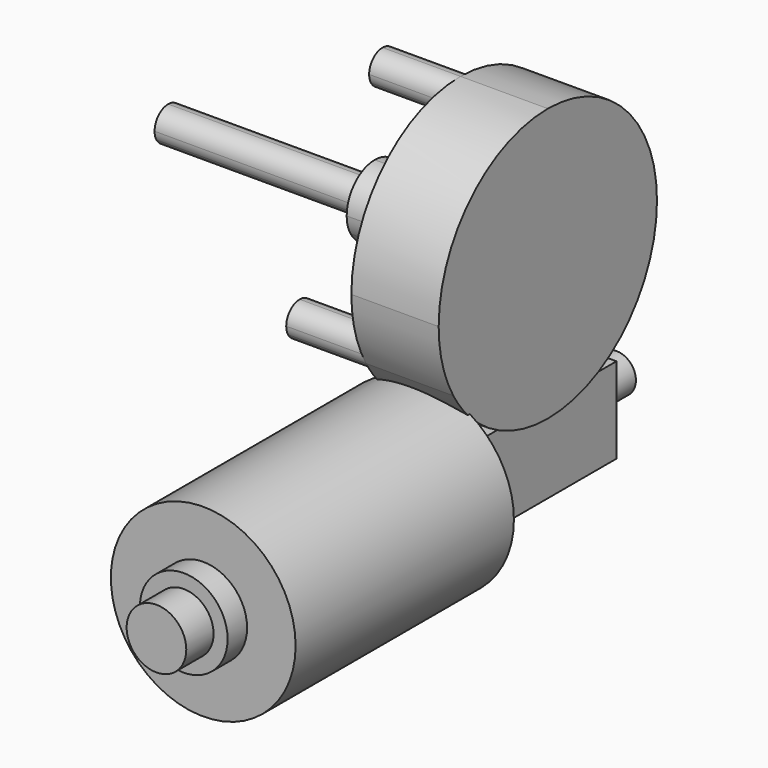
from build123d import *

# Parameters (mm, degrees)
F0_R      = 30.099
F0_R_2    = 14.2875
F0_R_3    = 9.7155
F1_DEPTH  = 88.9
F2_DEPTH  = 7.9375
F3_DEPTH  = 19.05
F4_W      = 25.4
F4_H      = 27.94
F4_R      = 6.35
F5_DEPTH  = 63.5
F6_DEPTH  = 79.375
F8_DEPTH  = 28.448
F9_DEPTH  = 27.94
F10_DEPTH = 95.25
F11_DEPTH = 25.4


# Not quite as in the source:
# - a length typed as a fraction of an inch, garbled in the dataset ("3 / 203.2 mm" for 3/8 in), is restored


with BuildPart() as f1:
    # F0 (on Front) → F1 (new body)
    with BuildSketch(Plane.XZ):
        Circle(F0_R)
        Circle(F0_R_2, mode=Mode.SUBTRACT)
        Circle(F0_R_2)
        Circle(F0_R_3, mode=Mode.SUBTRACT)
        Circle(F0_R_3)
    extrude(amount=-F1_DEPTH)

    # F0 (on Front) → F2 (join)
    with BuildSketch(Plane.XZ):
        Circle(F0_R_2)
        Circle(F0_R_3, mode=Mode.SUBTRACT)
    extrude(amount=F2_DEPTH)

    # F0 (on Front) → F3 (join)
    with BuildSketch(Plane.XZ):
        Circle(F0_R_3)
    extrude(amount=F3_DEPTH)

    # F4 (on face) → F5 (join)
    with BuildSketch(Plane(origin=(0, 88.9, 0), x_dir=(-1, 0, 0), z_dir=(0, 1, 0))):
        Rectangle(F4_W, F4_H)
        Circle(F4_R, mode=Mode.SUBTRACT)
    extrude(amount=F5_DEPTH)

    # F4 (on face) → F6 (join)
    with BuildSketch(Plane(origin=(0, 88.9, 0), x_dir=(-1, 0, 0), z_dir=(0, 1, 0))):
        Circle(F4_R)
    extrude(amount=F6_DEPTH)

    # F7 (on face) → F8 (join)
    with BuildSketch(Plane(origin=(-12.7, 0, 0), x_dir=(0, -1, 0), z_dir=(-1, 0, 0))):
        with BuildLine():
            Line((-120.65, 33.655), (-120.65, 13.97))
            Line((-120.65, 13.97), (-120.65, 11.43))
            ThreePointArc((-120.65, 11.43), (-98.425, 17.3851708018), (-82.1551708018, 33.655))
            ThreePointArc((-82.1551708018, 33.655), (-86.8845355318, 30.9245), (-91.6139002619, 33.655))
            Line((-91.6139002619, 33.655), (-120.65, 33.655))
        make_face()
        with BuildLine():
            Line((-120.65, 11.43), (-120.65, 13.97))
            Line((-120.65, 13.97), (-120.65, 33.655))
            Line((-120.65, 33.655), (-149.6860997381, 33.655))
            ThreePointArc((-149.6860997381, 33.655), (-154.4154644682, 30.9245), (-159.1448291982, 33.655))
            ThreePointArc((-159.1448291982, 33.655), (-142.875, 17.3851708018), (-120.65, 11.43))
        make_face()
        with BuildLine():
            Line((-156.5051837675, 35.179), (-159.1448291982, 33.655))
            Line((-159.1448291982, 33.655), (-149.6860997381, 33.655))
            ThreePointArc((-149.6860997381, 33.655), (-149.1405435308, 34.9720891947), (-148.9544644682, 36.3855))
            ThreePointArc((-148.9544644682, 36.3855), (-149.1405435308, 37.7989108053), (-149.6860997381, 39.116))
            Line((-149.6860997381, 39.116), (-152.3257451688, 37.592))
            ThreePointArc((-152.3257451688, 37.592), (-152.0846854493, 37.0100303558), (-152.0024644682, 36.3855))
            ThreePointArc((-152.0024644682, 36.3855), (-153.7909341123, 34.0547209812), (-156.5051837675, 35.179))
        make_face()
        with BuildLine():
            ThreePointArc((-154.4154644682, 41.8465), (-159.1448291982, 39.116), (-159.1448291982, 33.655))
            Line((-159.1448291982, 33.655), (-154.4154644682, 41.8465))
        make_face()
        with BuildLine():
            Line((-154.4154644682, 41.8465), (-159.1448291982, 33.655))
            Line((-159.1448291982, 33.655), (-156.5051837675, 35.179))
            ThreePointArc((-156.5051837675, 35.179), (-155.6219644682, 38.4752192993), (-152.3257451688, 37.592))
            Line((-152.3257451688, 37.592), (-149.6860997381, 39.116))
            ThreePointArc((-149.6860997381, 39.116), (-151.6849644682, 41.1148647301), (-154.4154644682, 41.8465))
        make_face()
        with BuildLine():
            ThreePointArc((-120.65, 100.33), (-159.1448291982, 78.105), (-159.1448291982, 33.655))
            ThreePointArc((-159.1448291982, 33.655), (-159.1448291982, 39.116), (-154.4154644682, 41.8465))
            Line((-154.4154644682, 41.8465), (-125.3793647301, 92.1385))
            ThreePointArc((-125.3793647301, 92.1385), (-125.3793647301, 97.5995), (-120.65, 100.33))
        make_face()
        with BuildLine():
            Line((-149.6860997381, 33.655), (-159.1448291982, 33.655))
            ThreePointArc((-159.1448291982, 33.655), (-154.4154644682, 30.9245), (-149.6860997381, 33.655))
        make_face()
        with BuildLine():
            ThreePointArc((-81.4235355318, 36.3855), (-81.6096145945, 34.9720891947), (-82.1551708018, 33.655))
            ThreePointArc((-82.1551708018, 33.655), (-77.7145970215, 44.3754934452), (-76.2, 55.88))
            ThreePointArc((-76.2, 55.88), (-89.2191035763, 87.3108964237), (-120.65, 100.33))
            ThreePointArc((-120.65, 100.33), (-116.7884898679, 98.7305101321), (-115.189, 94.869))
            ThreePointArc((-115.189, 94.869), (-115.3750790626, 93.4555891947), (-115.9206352699, 92.1385))
            Line((-115.9206352699, 92.1385), (-86.8845355318, 41.8465))
            ThreePointArc((-86.8845355318, 41.8465), (-83.0230253998, 40.2470101321), (-81.4235355318, 36.3855))
        make_face()
        with BuildLine():
            Line((-84.7948162325, 35.179), (-82.1551708018, 33.655))
            Line((-82.1551708018, 33.655), (-86.8845355318, 41.8465))
            ThreePointArc((-86.8845355318, 41.8465), (-89.6150355318, 41.1148647301), (-91.6139002619, 39.116))
            Line((-91.6139002619, 39.116), (-88.9742548312, 37.592))
            ThreePointArc((-88.9742548312, 37.592), (-86.260005176, 38.7162790188), (-84.4715355318, 36.3855))
            ThreePointArc((-84.4715355318, 36.3855), (-84.553756513, 35.7609696442), (-84.7948162325, 35.179))
        make_face()
        with BuildLine():
            ThreePointArc((-91.6139002619, 33.655), (-86.8845355318, 30.9245), (-82.1551708018, 33.655))
            Line((-82.1551708018, 33.655), (-91.6139002619, 33.655))
        make_face()
        with BuildLine():
            Line((-91.6139002619, 33.655), (-82.1551708018, 33.655))
            Line((-82.1551708018, 33.655), (-84.7948162325, 35.179))
            ThreePointArc((-84.7948162325, 35.179), (-88.0910355318, 34.2957807007), (-88.9742548312, 37.592))
            Line((-88.9742548312, 37.592), (-91.6139002619, 39.116))
            ThreePointArc((-91.6139002619, 39.116), (-92.3455355318, 36.3855), (-91.6139002619, 33.655))
        make_face()
        with BuildLine():
            Line((-86.8845355318, 41.8465), (-82.1551708018, 33.655))
            ThreePointArc((-82.1551708018, 33.655), (-81.6096145945, 34.9720891947), (-81.4235355318, 36.3855))
            ThreePointArc((-81.4235355318, 36.3855), (-83.0230253998, 40.2470101321), (-86.8845355318, 41.8465))
        make_face()
        with BuildLine():
            ThreePointArc((-115.189, 94.869), (-116.7884898679, 98.7305101321), (-120.65, 100.33))
            Line((-120.65, 100.33), (-115.9206352699, 92.1385))
            ThreePointArc((-115.9206352699, 92.1385), (-115.3750790626, 93.4555891947), (-115.189, 94.869))
        make_face()
        with BuildLine():
            Line((-120.65, 97.282), (-120.65, 100.33))
            Line((-120.65, 100.33), (-125.3793647301, 92.1385))
            ThreePointArc((-125.3793647301, 92.1385), (-123.3805, 90.1396352699), (-120.65, 89.408))
            Line((-120.65, 89.408), (-120.65, 92.456))
            ThreePointArc((-120.65, 92.456), (-123.063, 94.869), (-120.65, 97.282))
        make_face()
        with BuildLine():
            Line((-115.9206352699, 92.1385), (-120.65, 100.33))
            Line((-120.65, 100.33), (-120.65, 97.282))
            ThreePointArc((-120.65, 97.282), (-118.943751337, 96.575248663), (-118.237, 94.869))
            ThreePointArc((-118.237, 94.869), (-118.943751337, 93.162751337), (-120.65, 92.456))
            Line((-120.65, 92.456), (-120.65, 89.408))
            ThreePointArc((-120.65, 89.408), (-117.9195, 90.1396352699), (-115.9206352699, 92.1385))
        make_face()
        with BuildLine():
            Line((-125.3793647301, 92.1385), (-120.65, 100.33))
            ThreePointArc((-120.65, 100.33), (-125.3793647301, 97.5995), (-125.3793647301, 92.1385))
        make_face()
        with BuildLine():
            ThreePointArc((-120.65, 67.31), (-130.5486703653, 61.595), (-130.5486703653, 50.165))
            Line((-130.5486703653, 50.165), (-125.4343573432, 53.11775))
            ThreePointArc((-125.4343573432, 53.11775), (-125.4343573432, 58.64225), (-120.65, 61.4045))
            Line((-120.65, 61.4045), (-120.65, 67.31))
        make_face()
        with BuildLine():
            ThreePointArc((-130.5486703653, 50.165), (-126.365, 45.9813296347), (-120.65, 44.45))
            Line((-120.65, 44.45), (-120.65, 50.3555))
            ThreePointArc((-120.65, 50.3555), (-123.41225, 51.0956426568), (-125.4343573432, 53.11775))
            Line((-125.4343573432, 53.11775), (-130.5486703653, 50.165))
        make_face()
        with BuildLine():
            Line((-120.65, 50.3555), (-120.65, 44.45))
            ThreePointArc((-120.65, 44.45), (-114.935, 45.9813296347), (-110.7513296347, 50.165))
            Line((-110.7513296347, 50.165), (-115.8656426568, 53.11775))
            ThreePointArc((-115.8656426568, 53.11775), (-117.88775, 51.0956426568), (-120.65, 50.3555))
        make_face()
        with BuildLine():
            Line((-115.8656426568, 53.11775), (-110.7513296347, 50.165))
            ThreePointArc((-110.7513296347, 50.165), (-109.6094678055, 52.9216983145), (-109.22, 55.88))
            ThreePointArc((-109.22, 55.88), (-112.567769491, 63.962230509), (-120.65, 67.31))
            Line((-120.65, 67.31), (-120.65, 61.4045))
            ThreePointArc((-120.65, 61.4045), (-116.7435885873, 59.7864114127), (-115.1255, 55.88))
            ThreePointArc((-115.1255, 55.88), (-115.3137427727, 54.4501541853), (-115.8656426568, 53.11775))
        make_face()
        with BuildLine():
            Line((-125.4343573432, 53.11775), (-120.65, 55.88))
            Line((-120.65, 55.88), (-120.65, 61.4045))
            ThreePointArc((-120.65, 61.4045), (-125.4343573432, 58.64225), (-125.4343573432, 53.11775))
        make_face()
        with BuildLine():
            ThreePointArc((-125.4343573432, 53.11775), (-123.41225, 51.0956426568), (-120.65, 50.3555))
            Line((-120.65, 50.3555), (-120.65, 55.88))
            Line((-120.65, 55.88), (-125.4343573432, 53.11775))
        make_face()
        with BuildLine():
            Line((-120.65, 55.88), (-120.65, 50.3555))
            ThreePointArc((-120.65, 50.3555), (-117.88775, 51.0956426568), (-115.8656426568, 53.11775))
            Line((-115.8656426568, 53.11775), (-120.65, 55.88))
        make_face()
        with BuildLine():
            Line((-120.65, 61.4045), (-120.65, 55.88))
            Line((-120.65, 55.88), (-115.8656426568, 53.11775))
            ThreePointArc((-115.8656426568, 53.11775), (-115.3137427727, 54.4501541853), (-115.1255, 55.88))
            ThreePointArc((-115.1255, 55.88), (-116.7435885873, 59.7864114127), (-120.65, 61.4045))
        make_face()
        with BuildLine():
            ThreePointArc((-109.22, 55.88), (-109.6094678055, 52.9216983145), (-110.7513296347, 50.165))
            Line((-110.7513296347, 50.165), (-91.6139002619, 39.116))
            ThreePointArc((-91.6139002619, 39.116), (-89.6150355318, 41.1148647301), (-86.8845355318, 41.8465))
            Line((-86.8845355318, 41.8465), (-115.9206352699, 92.1385))
            ThreePointArc((-115.9206352699, 92.1385), (-117.9195, 90.1396352699), (-120.65, 89.408))
            Line((-120.65, 89.408), (-120.65, 67.31))
            ThreePointArc((-120.65, 67.31), (-112.567769491, 63.962230509), (-109.22, 55.88))
        make_face()
        with BuildLine():
            Line((-149.6860997381, 39.116), (-130.5486703653, 50.165))
            ThreePointArc((-130.5486703653, 50.165), (-130.5486703653, 61.595), (-120.65, 67.31))
            Line((-120.65, 67.31), (-120.65, 89.408))
            ThreePointArc((-120.65, 89.408), (-123.3805, 90.1396352699), (-125.3793647301, 92.1385))
            Line((-125.3793647301, 92.1385), (-154.4154644682, 41.8465))
            ThreePointArc((-154.4154644682, 41.8465), (-151.6849644682, 41.1148647301), (-149.6860997381, 39.116))
        make_face()
        with BuildLine():
            Line((-149.6860997381, 33.655), (-120.65, 33.655))
            Line((-120.65, 33.655), (-120.65, 44.45))
            ThreePointArc((-120.65, 44.45), (-126.365, 45.9813296347), (-130.5486703653, 50.165))
            Line((-130.5486703653, 50.165), (-149.6860997381, 39.116))
            ThreePointArc((-149.6860997381, 39.116), (-149.1405435308, 37.7989108053), (-148.9544644682, 36.3855))
            ThreePointArc((-148.9544644682, 36.3855), (-149.1405435308, 34.9720891947), (-149.6860997381, 33.655))
        make_face()
        with BuildLine():
            Line((-120.65, 44.45), (-120.65, 33.655))
            Line((-120.65, 33.655), (-91.6139002619, 33.655))
            ThreePointArc((-91.6139002619, 33.655), (-92.3455355318, 36.3855), (-91.6139002619, 39.116))
            Line((-91.6139002619, 39.116), (-110.7513296347, 50.165))
            ThreePointArc((-110.7513296347, 50.165), (-114.935, 45.9813296347), (-120.65, 44.45))
        make_face()
        with BuildLine():
            ThreePointArc((-152.3257451688, 37.592), (-155.6219644682, 38.4752192993), (-156.5051837675, 35.179))
            Line((-156.5051837675, 35.179), (-154.4154644682, 36.3855))
            Line((-154.4154644682, 36.3855), (-152.3257451688, 37.592))
        make_face()
        with BuildLine():
            Line((-154.4154644682, 36.3855), (-156.5051837675, 35.179))
            ThreePointArc((-156.5051837675, 35.179), (-153.7909341123, 34.0547209812), (-152.0024644682, 36.3855))
            ThreePointArc((-152.0024644682, 36.3855), (-152.0846854493, 37.0100303558), (-152.3257451688, 37.592))
            Line((-152.3257451688, 37.592), (-154.4154644682, 36.3855))
        make_face()
        with BuildLine():
            Line((-86.8845355318, 36.3855), (-84.7948162325, 35.179))
            ThreePointArc((-84.7948162325, 35.179), (-84.553756513, 35.7609696442), (-84.4715355318, 36.3855))
            ThreePointArc((-84.4715355318, 36.3855), (-86.260005176, 38.7162790188), (-88.9742548312, 37.592))
            Line((-88.9742548312, 37.592), (-86.8845355318, 36.3855))
        make_face()
        with BuildLine():
            ThreePointArc((-88.9742548312, 37.592), (-88.0910355318, 34.2957807007), (-84.7948162325, 35.179))
            Line((-84.7948162325, 35.179), (-86.8845355318, 36.3855))
            Line((-86.8845355318, 36.3855), (-88.9742548312, 37.592))
        make_face()
        with BuildLine():
            Line((-120.65, 94.869), (-120.65, 97.282))
            ThreePointArc((-120.65, 97.282), (-123.063, 94.869), (-120.65, 92.456))
            Line((-120.65, 92.456), (-120.65, 94.869))
        make_face()
        with BuildLine():
            ThreePointArc((-118.237, 94.869), (-118.943751337, 96.575248663), (-120.65, 97.282))
            Line((-120.65, 97.282), (-120.65, 94.869))
            Line((-120.65, 94.869), (-120.65, 92.456))
            ThreePointArc((-120.65, 92.456), (-118.943751337, 93.162751337), (-118.237, 94.869))
        make_face()
    extrude(amount=-F8_DEPTH)

    # F7 (on face) → F9 (join)
    with BuildSketch(Plane(origin=(-12.7, 0, 0), x_dir=(0, -1, 0), z_dir=(-1, 0, 0))):
        with BuildLine():
            ThreePointArc((-120.65, 67.31), (-130.5486703653, 61.595), (-130.5486703653, 50.165))
            Line((-130.5486703653, 50.165), (-125.4343573432, 53.11775))
            ThreePointArc((-125.4343573432, 53.11775), (-125.4343573432, 58.64225), (-120.65, 61.4045))
            Line((-120.65, 61.4045), (-120.65, 67.31))
        make_face()
        with BuildLine():
            ThreePointArc((-130.5486703653, 50.165), (-126.365, 45.9813296347), (-120.65, 44.45))
            Line((-120.65, 44.45), (-120.65, 50.3555))
            ThreePointArc((-120.65, 50.3555), (-123.41225, 51.0956426568), (-125.4343573432, 53.11775))
            Line((-125.4343573432, 53.11775), (-130.5486703653, 50.165))
        make_face()
        with BuildLine():
            Line((-120.65, 50.3555), (-120.65, 44.45))
            ThreePointArc((-120.65, 44.45), (-114.935, 45.9813296347), (-110.7513296347, 50.165))
            Line((-110.7513296347, 50.165), (-115.8656426568, 53.11775))
            ThreePointArc((-115.8656426568, 53.11775), (-117.88775, 51.0956426568), (-120.65, 50.3555))
        make_face()
        with BuildLine():
            Line((-115.8656426568, 53.11775), (-110.7513296347, 50.165))
            ThreePointArc((-110.7513296347, 50.165), (-109.6094678055, 52.9216983145), (-109.22, 55.88))
            ThreePointArc((-109.22, 55.88), (-112.567769491, 63.962230509), (-120.65, 67.31))
            Line((-120.65, 67.31), (-120.65, 61.4045))
            ThreePointArc((-120.65, 61.4045), (-116.7435885873, 59.7864114127), (-115.1255, 55.88))
            ThreePointArc((-115.1255, 55.88), (-115.3137427727, 54.4501541853), (-115.8656426568, 53.11775))
        make_face()
        with BuildLine():
            Line((-125.4343573432, 53.11775), (-120.65, 55.88))
            Line((-120.65, 55.88), (-120.65, 61.4045))
            ThreePointArc((-120.65, 61.4045), (-125.4343573432, 58.64225), (-125.4343573432, 53.11775))
        make_face()
        with BuildLine():
            ThreePointArc((-125.4343573432, 53.11775), (-123.41225, 51.0956426568), (-120.65, 50.3555))
            Line((-120.65, 50.3555), (-120.65, 55.88))
            Line((-120.65, 55.88), (-125.4343573432, 53.11775))
        make_face()
        with BuildLine():
            Line((-120.65, 55.88), (-120.65, 50.3555))
            ThreePointArc((-120.65, 50.3555), (-117.88775, 51.0956426568), (-115.8656426568, 53.11775))
            Line((-115.8656426568, 53.11775), (-120.65, 55.88))
        make_face()
        with BuildLine():
            Line((-120.65, 61.4045), (-120.65, 55.88))
            Line((-120.65, 55.88), (-115.8656426568, 53.11775))
            ThreePointArc((-115.8656426568, 53.11775), (-115.3137427727, 54.4501541853), (-115.1255, 55.88))
            ThreePointArc((-115.1255, 55.88), (-116.7435885873, 59.7864114127), (-120.65, 61.4045))
        make_face()
    extrude(amount=F9_DEPTH)

    # F7 (on face) → F10 (join)
    with BuildSketch(Plane(origin=(-12.7, 0, 0), x_dir=(0, -1, 0), z_dir=(-1, 0, 0))):
        with BuildLine():
            Line((-125.4343573432, 53.11775), (-120.65, 55.88))
            Line((-120.65, 55.88), (-120.65, 61.4045))
            ThreePointArc((-120.65, 61.4045), (-125.4343573432, 58.64225), (-125.4343573432, 53.11775))
        make_face()
        with BuildLine():
            ThreePointArc((-125.4343573432, 53.11775), (-123.41225, 51.0956426568), (-120.65, 50.3555))
            Line((-120.65, 50.3555), (-120.65, 55.88))
            Line((-120.65, 55.88), (-125.4343573432, 53.11775))
        make_face()
        with BuildLine():
            Line((-120.65, 55.88), (-120.65, 50.3555))
            ThreePointArc((-120.65, 50.3555), (-117.88775, 51.0956426568), (-115.8656426568, 53.11775))
            Line((-115.8656426568, 53.11775), (-120.65, 55.88))
        make_face()
        with BuildLine():
            Line((-120.65, 61.4045), (-120.65, 55.88))
            Line((-120.65, 55.88), (-115.8656426568, 53.11775))
            ThreePointArc((-115.8656426568, 53.11775), (-115.3137427727, 54.4501541853), (-115.1255, 55.88))
            ThreePointArc((-115.1255, 55.88), (-116.7435885873, 59.7864114127), (-120.65, 61.4045))
        make_face()
    extrude(amount=F10_DEPTH)

    # F7 (on face) → F11 (join)
    with BuildSketch(Plane(origin=(-12.7, 0, 0), x_dir=(0, -1, 0), z_dir=(-1, 0, 0))):
        with BuildLine():
            ThreePointArc((-154.4154644682, 41.8465), (-159.1448291982, 39.116), (-159.1448291982, 33.655))
            Line((-159.1448291982, 33.655), (-154.4154644682, 41.8465))
        make_face()
        with BuildLine():
            ThreePointArc((-159.1448291982, 33.655), (-154.4154644682, 30.9245), (-149.6860997381, 33.655))
            Line((-149.6860997381, 33.655), (-159.1448291982, 33.655))
        make_face()
        with BuildLine():
            Line((-82.1551708018, 33.655), (-91.6139002619, 33.655))
            ThreePointArc((-91.6139002619, 33.655), (-86.8845355318, 30.9245), (-82.1551708018, 33.655))
        make_face()
        with BuildLine():
            Line((-86.8845355318, 41.8465), (-82.1551708018, 33.655))
            ThreePointArc((-82.1551708018, 33.655), (-81.6096145945, 34.9720891947), (-81.4235355318, 36.3855))
            ThreePointArc((-81.4235355318, 36.3855), (-83.0230253998, 40.2470101321), (-86.8845355318, 41.8465))
        make_face()
        with BuildLine():
            ThreePointArc((-115.189, 94.869), (-116.7884898679, 98.7305101321), (-120.65, 100.33))
            Line((-120.65, 100.33), (-115.9206352699, 92.1385))
            ThreePointArc((-115.9206352699, 92.1385), (-115.3750790626, 93.4555891947), (-115.189, 94.869))
        make_face()
        with BuildLine():
            Line((-125.3793647301, 92.1385), (-120.65, 100.33))
            ThreePointArc((-120.65, 100.33), (-125.3793647301, 97.5995), (-125.3793647301, 92.1385))
        make_face()
        with BuildLine():
            Line((-84.7948162325, 35.179), (-82.1551708018, 33.655))
            Line((-82.1551708018, 33.655), (-86.8845355318, 41.8465))
            ThreePointArc((-86.8845355318, 41.8465), (-89.6150355318, 41.1148647301), (-91.6139002619, 39.116))
            Line((-91.6139002619, 39.116), (-88.9742548312, 37.592))
            ThreePointArc((-88.9742548312, 37.592), (-86.260005176, 38.7162790188), (-84.4715355318, 36.3855))
            ThreePointArc((-84.4715355318, 36.3855), (-84.553756513, 35.7609696442), (-84.7948162325, 35.179))
        make_face()
        with BuildLine():
            ThreePointArc((-91.6139002619, 39.116), (-92.3455355318, 36.3855), (-91.6139002619, 33.655))
            Line((-91.6139002619, 33.655), (-82.1551708018, 33.655))
            Line((-82.1551708018, 33.655), (-84.7948162325, 35.179))
            ThreePointArc((-84.7948162325, 35.179), (-88.0910355318, 34.2957807007), (-88.9742548312, 37.592))
            Line((-88.9742548312, 37.592), (-91.6139002619, 39.116))
        make_face()
        with BuildLine():
            Line((-159.1448291982, 33.655), (-149.6860997381, 33.655))
            ThreePointArc((-149.6860997381, 33.655), (-149.1405435308, 34.9720891947), (-148.9544644682, 36.3855))
            ThreePointArc((-148.9544644682, 36.3855), (-149.1405435308, 37.7989108053), (-149.6860997381, 39.116))
            Line((-149.6860997381, 39.116), (-152.3257451688, 37.592))
            ThreePointArc((-152.3257451688, 37.592), (-152.0846854493, 37.0100303558), (-152.0024644682, 36.3855))
            ThreePointArc((-152.0024644682, 36.3855), (-153.7909341123, 34.0547209812), (-156.5051837675, 35.179))
            Line((-156.5051837675, 35.179), (-159.1448291982, 33.655))
        make_face()
        with BuildLine():
            Line((-154.4154644682, 41.8465), (-159.1448291982, 33.655))
            Line((-159.1448291982, 33.655), (-156.5051837675, 35.179))
            ThreePointArc((-156.5051837675, 35.179), (-155.6219644682, 38.4752192993), (-152.3257451688, 37.592))
            Line((-152.3257451688, 37.592), (-149.6860997381, 39.116))
            ThreePointArc((-149.6860997381, 39.116), (-151.6849644682, 41.1148647301), (-154.4154644682, 41.8465))
        make_face()
        with BuildLine():
            Line((-115.9206352699, 92.1385), (-120.65, 100.33))
            Line((-120.65, 100.33), (-120.65, 97.282))
            ThreePointArc((-120.65, 97.282), (-118.943751337, 96.575248663), (-118.237, 94.869))
            ThreePointArc((-118.237, 94.869), (-118.943751337, 93.162751337), (-120.65, 92.456))
            Line((-120.65, 92.456), (-120.65, 89.408))
            ThreePointArc((-120.65, 89.408), (-117.9195, 90.1396352699), (-115.9206352699, 92.1385))
        make_face()
        with BuildLine():
            Line((-120.65, 97.282), (-120.65, 100.33))
            Line((-120.65, 100.33), (-125.3793647301, 92.1385))
            ThreePointArc((-125.3793647301, 92.1385), (-123.3805, 90.1396352699), (-120.65, 89.408))
            Line((-120.65, 89.408), (-120.65, 92.456))
            ThreePointArc((-120.65, 92.456), (-123.063, 94.869), (-120.65, 97.282))
        make_face()
    extrude(amount=F11_DEPTH)


solid = f1.part
